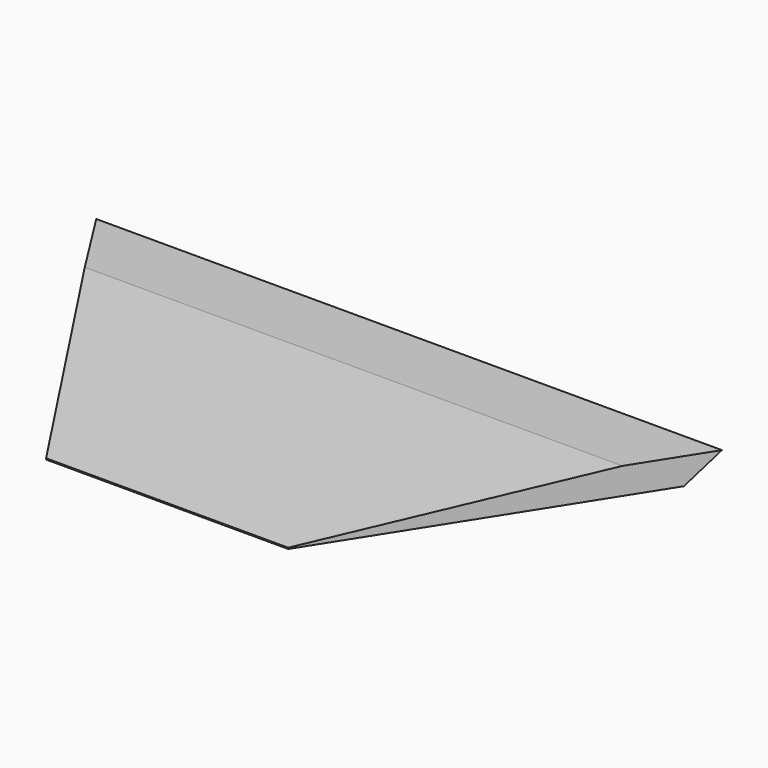
from build123d import *

# Parameters (mm, degrees)
F1_DEPTH = 6.35
F2_SIZE  = 6.34999
F3_SIZE2 = 6.0705106322
F3_SIZE  = 55.88


# Not quite as in the source:
# - a fillet or chamfer is up to 0.001 mm smaller than in the source, because OpenCascade refuses the exact size


with BuildPart() as f1:
    # F0 (on Top) → F1 (new body)
    with BuildSketch(Plane.XY):
        Polygon((75, 225), (-75, 225), (-29.020415619, 152.489066124), (29.020415619, 152.489066124), align=None)
    extrude(amount=F1_DEPTH)

    # F2 (size 6.35 in the source; OpenCascade refuses exactly that, so slightly less here)
    f2_edges = [f1.edges().sort_by_distance(p)[0] for p in [
        (0, 225, 0),
    ]]
    chamfer(f2_edges, length=F2_SIZE)

    # F3
    f3_edges = [f1.edges().sort_by_distance(p)[0] for p in [
        (0, 152.489066, 6.35),
    ]]
    f3_side = f1.faces().sort_by_distance((0, 194.086469, 6.35))[0]
    chamfer(f3_edges, length=F3_SIZE, length2=F3_SIZE2, reference=f3_side)


solid = f1.part
